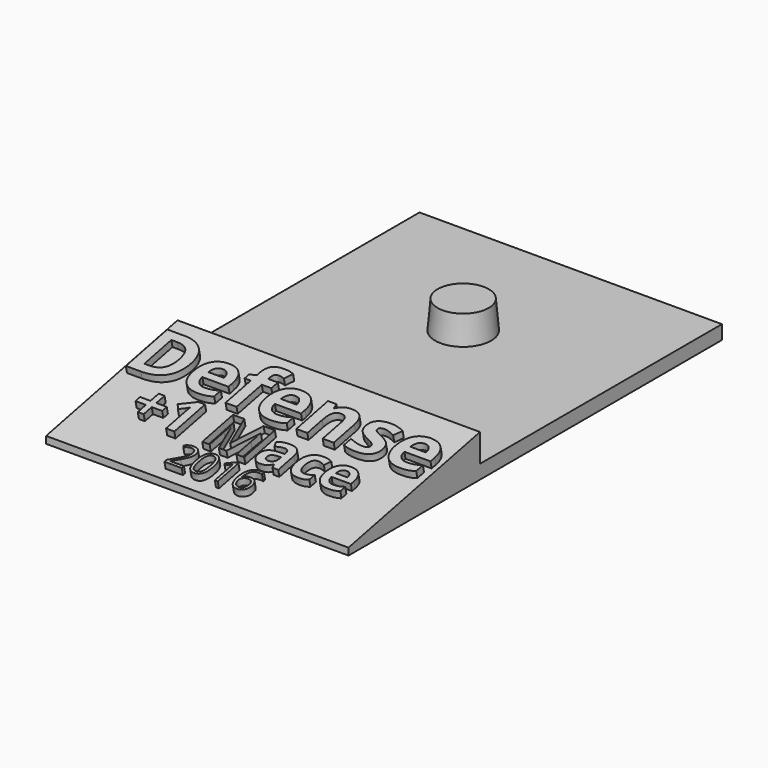
from build123d import *

# Parameters (mm, degrees)
F1_DEPTH       = 34.29
F2_R           = 6.35
F3_DEPTH       = 6.35
F3_TAPER       = 5
F4_TEXT_SIZE   = 16.8255769378
F4_TEXT_SIZE_2 = 12.4657796864
F4_TEXT_SIZE_3 = 8.3822240315
F5_DEPTH       = 1.5875


# Not quite as in the source:
# - Text() gives the source's letters only with a copy of the font that has no kerning and outlines rounded to 1/6400 em; it was checked with that copy


with BuildPart() as f1:
    # F0 (on Right) → F1 (new body, symmetric)
    with BuildSketch(Plane.YZ):
        Polygon((-105.8440053369, 0), (0, 0), (0, 3.175), (-68.58, 3.175), (-68.58, 9.525), (-105.8440053369, 1.5875), align=None)
    extrude(amount=F1_DEPTH, both=True)

    # F2 (on face) → F3 (join)
    with BuildSketch(Plane.XY.offset(3.175)):
        with Locations((0, -30.48)):
            Circle(F2_R)
    extrude(amount=F3_DEPTH, taper=F3_TAPER)

    # F4 (on face) → F5 (join)
    with BuildSketch(Plane(origin=(0, -4.9173961113, 23.085590543), x_dir=(1, 0, 0), z_dir=(0, -0.2083333333, 0.9780578829))):
        with Locations((-34.29, -81.6646093236)):
            Text('Defense', F4_TEXT_SIZE, font='Open Sans', font_style=FontStyle.BOLD, text_align=(TextAlign.LEFT, TextAlign.BOTTOM))
        with Locations((-25.4, -92.7131476504)):
            Text('+1 Mace', F4_TEXT_SIZE_2, font='Open Sans', font_style=FontStyle.BOLD, text_align=(TextAlign.LEFT, TextAlign.BOTTOM))
        with Locations((-9.652, -100.5707048135)):
            Text('2016', F4_TEXT_SIZE_3, font='Open Sans', text_align=(TextAlign.LEFT, TextAlign.BOTTOM))
    extrude(amount=F5_DEPTH)


solid = f1.part
